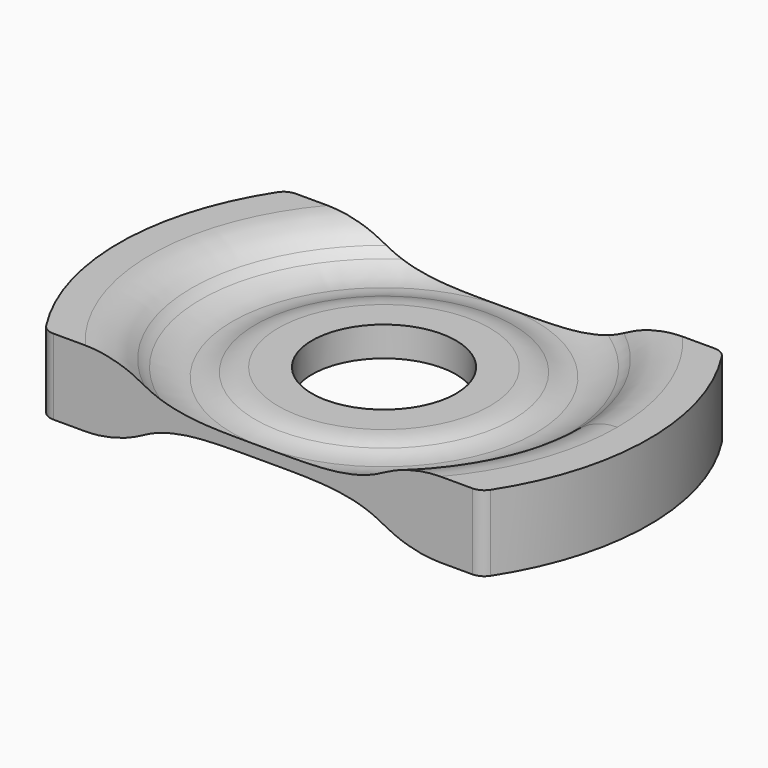
from build123d import *

# Parameters (mm, degrees)
F0_R            = 6.035
F1_DEPTH        = 3.175
F3_COPIES_COUNT = 2
F4_T3_ANGLE     = 67.6677552602
F4_T6_ANGLE     = 67.6677552602
F4_T9_ANGLE     = 135.3490310549
F4_T18_ANGLE    = 135.3490310549
F4_T21_ANGLE    = 67.6677552602
F4_T24_ANGLE    = 67.6677552602
F5_R            = 1.27


# Not quite as in the source:
# - a fillet or chamfer that OpenCascade refuses, or shapes differently, is made with other operations: its cross-section is extruded or revolved along the edge and cut away or added
# - a pattern or mirror of a feature is missing from the dataset's text; its kind, count and spacing are read off the source's solid


with BuildPart() as f1:
    # F0 (on Top) → F1 (new body, symmetric)
    with BuildSketch(Plane.XY):
        with BuildLine():
            Line((18.2389864028, 12.7), (-18.2389864028, 12.7))
            ThreePointArc((-18.2389864028, 12.7), (-22.225, 0), (-18.2389864028, -12.7))
            Line((-18.2389864028, -12.7), (18.2389864028, -12.7))
            ThreePointArc((18.2389864028, -12.7), (22.225, 0), (18.2389864028, 12.7))
        make_face()
        Circle(F0_R, mode=Mode.SUBTRACT)
    extrude(amount=F1_DEPTH, both=True)

    # F2 (on Front) → F3 (revolve, cut)
    with BuildSketch(Plane.XZ):
        with BuildLine():
            ThreePointArc((15.3565955658, 1.25), (17.1329395143, 3.0989826153), (17.78, 5.58))
            ThreePointArc((17.78, 5.58), (13.844578608, 10.5293777195), (8.1357717283, 7.8102960081))
            ThreePointArc((8.1357717283, 7.8102960081), (7.8220449826, 4.1615660577), (10.0434044342, 1.25))
            Line((10.0434044342, 1.25), (12.7, 1.25))
            Line((12.7, 1.25), (15.3565955658, 1.25))
        make_face()
        with BuildLine():
            ThreePointArc((10.0434044342, 1.25), (7.8220449826, 4.1615660577), (8.1357717283, 7.8102960081))
            Line((8.1357717283, 7.8102960081), (0, 7.8102960081))
            Line((0, 7.8102960081), (0, 1.25))
            Line((0, 1.25), (10.0434044342, 1.25))
        make_face()
        with BuildLine():
            ThreePointArc((12.7, 0.5), (14.0802173742, 0.6910941919), (15.3565955658, 1.25))
            Line((15.3565955658, 1.25), (12.7, 1.25))
            Line((12.7, 1.25), (12.7, 0.5))
        make_face()
        with BuildLine():
            Line((12.7, 1.25), (10.0434044342, 1.25))
            ThreePointArc((10.0434044342, 1.25), (11.3197826258, 0.6910941919), (12.7, 0.5))
            Line((12.7, 0.5), (12.7, 1.25))
        make_face()
    f3 = revolve(axis=Axis((0, 0, 0), (0, 0, -1)), mode=Mode.SUBTRACT)

    # F3_copies: F3 ×2 about axis
    f3_copies_axis = Axis((0, 0, 0), (1, 0, 0))
    for i in range(1, F3_COPIES_COUNT):
        add(f3.rotate(f3_copies_axis, i * 360 / F3_COPIES_COUNT), mode=Mode.SUBTRACT)

    # F4: fillet of radius 5.08 on 9 edges, made by hand


with BuildPart() as f4_tool1:
    # F4_s2 → F4_t3 (revolve)
    with BuildSketch(Plane(origin=(0, 0, 0), x_dir=(0, 0, 1), z_dir=(-0.9249960227, -0.379976786, 0))):
        with BuildLine():
            ThreePointArc((1.8375, -16.1351264533), (2.828830373, -17.7270898644), (3.175, -19.5702529066))
            Line((3.175, -19.5702529066), (3.175, -17.1746368568))
            ThreePointArc((3.175, -17.1746368568), (2.4626157548, -16.7110242417), (1.8375, -16.1351264533))
        make_face()
    revolve(axis=Axis((0, 0, 3.175), (0, 0, 1)), revolution_arc=F4_T3_ANGLE)


with BuildPart() as f4_tool4:
    # F4_s5 → F4_t6 (revolve)
    with BuildSketch(Plane.XZ):
        with BuildLine():
            ThreePointArc((16.1351264533, 1.8375), (17.7270898644, 2.828830373), (19.5702529066, 3.175))
            Line((19.5702529066, 3.175), (17.1746368568, 3.175))
            ThreePointArc((17.1746368568, 3.175), (16.7110242417, 2.4626157548), (16.1351264533, 1.8375))
        make_face()
    revolve(axis=Axis((0, 0, 3.175), (0, 0, 1)), revolution_arc=F4_T6_ANGLE)


with BuildPart() as f4_tool7:
    # F4_s8 → F4_t9 (revolve)
    with BuildSketch(Plane(origin=(0, 0, 0), x_dir=(0, 0, 1), z_dir=(0.9250408493, 0.3798676441, 0))):
        with BuildLine():
            ThreePointArc((1.8375, -16.1351264533), (2.828830373, -17.7270898644), (3.175, -19.5702529066))
            Line((3.175, -19.5702529066), (3.175, -17.1746368568))
            ThreePointArc((3.175, -17.1746368568), (2.4626157548, -16.7110242417), (1.8375, -16.1351264533))
        make_face()
    revolve(axis=Axis((0, 0, 3.175), (0, 0, 1)), revolution_arc=F4_T9_ANGLE)


with BuildPart() as f4_tool10:
    # F4_s11 → F4_t12 (revolve)
    with BuildSketch(Plane.XZ):
        with BuildLine():
            ThreePointArc((10.7844387246, 0.875), (9.8448385139, 1.1553685922), (8.8688774491, 1.25))
            Line((8.8688774491, 1.25), (10.0434044342, 1.25))
            ThreePointArc((10.0434044342, 1.25), (10.4062452626, 1.0473308962), (10.7844387246, 0.875))
        make_face()
    revolve(axis=Axis((0, 0, 1.25), (0, 0, -1)))


with BuildPart() as f4_tool13:
    # F4_s14 → F4_t15 (revolve)
    with BuildSketch(Plane.XZ):
        with BuildLine():
            ThreePointArc((8.8688774491, -1.25), (9.8448385139, -1.1553685922), (10.7844387245, -0.875))
            ThreePointArc((10.7844387245, -0.875), (10.4062452626, -1.0473308962), (10.0434044342, -1.25))
            Line((10.0434044342, -1.25), (8.8688774491, -1.25))
        make_face()
    revolve(axis=Axis((0, 0, -1.25), (0, 0, 1)))


with BuildPart() as f4_tool16:
    # F4_s17 → F4_t18 (revolve)
    with BuildSketch(Plane(origin=(0, 0, 0), x_dir=(0, 0, 1), z_dir=(0.9250408493, -0.3798676441, 0))):
        with BuildLine():
            ThreePointArc((-3.175, 19.5702529066), (-2.828830373, 17.7270898644), (-1.8375, 16.1351264533))
            ThreePointArc((-1.8375, 16.1351264533), (-2.4626157548, 16.7110242417), (-3.175, 17.1746368568))
            Line((-3.175, 17.1746368568), (-3.175, 19.5702529066))
        make_face()
    revolve(axis=Axis((0, 0, -3.175), (0, 0, -1)), revolution_arc=F4_T18_ANGLE)


with BuildPart() as f4_tool19:
    # F4_s20 → F4_t21 (revolve)
    with BuildSketch(Plane.XZ):
        with BuildLine():
            ThreePointArc((16.1351264533, -1.8375), (17.7270898644, -2.828830373), (19.5702529066, -3.175))
            Line((19.5702529066, -3.175), (17.1746368568, -3.175))
            ThreePointArc((17.1746368568, -3.175), (16.7110242417, -2.4626157548), (16.1351264533, -1.8375))
        make_face()
    revolve(axis=Axis((0, 0, -3.175), (0, 0, -1)), revolution_arc=F4_T21_ANGLE)


with BuildPart() as f4_tool22:
    # F4_s23 → F4_t24 (revolve)
    with BuildSketch(Plane(origin=(0, 0, 0), x_dir=(0, 0, 1), z_dir=(-0.9249960227, 0.379976786, 0))):
        with BuildLine():
            ThreePointArc((-1.8375, 16.1351264533), (-2.828830373, 17.7270898644), (-3.175, 19.5702529066))
            Line((-3.175, 19.5702529066), (-3.175, 17.1746368568))
            ThreePointArc((-3.175, 17.1746368568), (-2.4626157548, 16.7110242417), (-1.8375, 16.1351264533))
        make_face()
    revolve(axis=Axis((0, 0, -3.175), (0, 0, -1)), revolution_arc=F4_T24_ANGLE)


with BuildPart() as f1_1:
    add(f1.part)

    # F4_t25: cut F4_tool1, F4_tool4, F4_tool7, F4_tool10, F4_tool13, F4_tool16, F4_tool19, F4_tool22
    add([f4_tool1.part, f4_tool4.part, f4_tool7.part, f4_tool10.part, f4_tool13.part, f4_tool16.part, f4_tool19.part, f4_tool22.part], mode=Mode.SUBTRACT)

    # F5
    f5_edges = [f1_1.edges().sort_by_distance(p)[0] for p in [
        (-18.238986, -12.7, 0),
        (-18.238986, 12.7, 0),
        (18.238986, 12.7, 0),
        (18.238986, -12.7, 0),
    ]]
    fillet(f5_edges, radius=F5_R)


solid = f1_1.part
